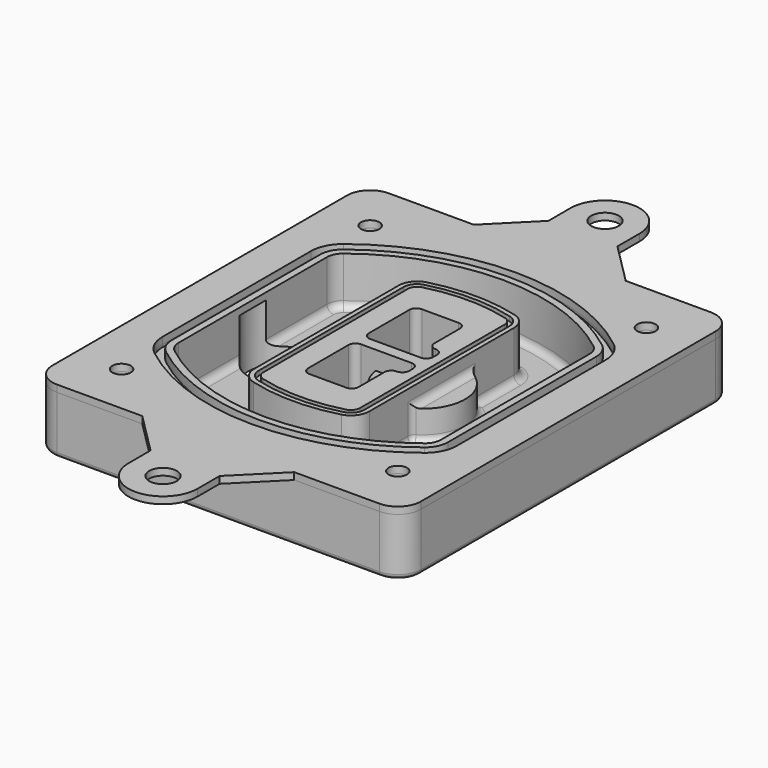
from build123d import *

# Parameters (mm, degrees)
F0_R      = 4
F1_DEPTH  = 25
F2_DEPTH  = 3
F3_DEPTH  = 1
F4_DEPTH  = 18
F6_DEPTH  = 21
F7_DEPTH  = 2
F9_DEPTH  = 20
F10_DEPTH = 16
F11_DEPTH = 25
F8_R      = 6
F8_R_2    = 4
F12_DEPTH = 6
F14_DEPTH = 9
F15_R     = 3
F16_R     = 2
F0_R_2    = 6
F17_DEPTH = 3


with BuildPart() as f1:
    # F0 (on Top) → F1 (new body)
    with BuildSketch(Plane.XY):
        with BuildLine():
            ThreePointArc((-80, -80), (-77.0710678119, -87.0710678119), (-70, -90))
            Line((-70, -90), (-33, -90))
            Line((-33, -90), (33, -90))
            Line((33, -90), (70, -90))
            ThreePointArc((70, -90), (77.0710678119, -87.0710678119), (80, -80))
            Line((80, -80), (80, 80))
            ThreePointArc((80, 80), (77.0710678119, 87.0710678119), (70, 90))
            Line((70, 90), (33, 90))
            Line((33, 90), (-33, 90))
            Line((-33, 90), (-70, 90))
            ThreePointArc((-70, 90), (-77.0710678119, 87.0710678119), (-80, 80))
            Line((-80, 80), (-80, -80))
        make_face()
        with Locations((-60, -67.5)):
            Circle(F0_R, mode=Mode.SUBTRACT)
        with Locations((60, -67.5)):
            Circle(F0_R, mode=Mode.SUBTRACT)
        with Locations((-60, 67.5)):
            Circle(F0_R, mode=Mode.SUBTRACT)
        with BuildLine():
            ThreePointArc((-64, 40.2934422872), (-62.5820384798, 46.4328484224), (-58.6153846154, 51.3286200352))
            ThreePointArc((-58.6153846154, 51.3286200352), (0, 71.5), (58.6153846154, 51.3286200352))
            ThreePointArc((58.6153846154, 51.3286200352), (62.5820384798, 46.4328484224), (64, 40.2934422872))
            Line((64, 40.2934422872), (64, -40.2934422872))
            ThreePointArc((64, -40.2934422872), (62.5820384798, -46.4328484224), (58.6153846154, -51.3286200352))
            ThreePointArc((58.6153846154, -51.3286200352), (0, -71.5), (-58.6153846154, -51.3286200352))
            ThreePointArc((-58.6153846154, -51.3286200352), (-62.5820384798, -46.4328484224), (-64, -40.2934422872))
            Line((-64, -40.2934422872), (-64, 40.2934422872))
        make_face(mode=Mode.SUBTRACT)
        with Locations((60, 67.5)):
            Circle(F0_R, mode=Mode.SUBTRACT)
        with BuildLine():
            ThreePointArc((58.6153846154, 51.3286200352), (0, 71.5), (-58.6153846154, 51.3286200352))
            ThreePointArc((-58.6153846154, 51.3286200352), (-62.5820384798, 46.4328484224), (-64, 40.2934422872))
            Line((-64, 40.2934422872), (-64, -40.2934422872))
            ThreePointArc((-64, -40.2934422872), (-62.5820384798, -46.4328484224), (-58.6153846154, -51.3286200352))
            ThreePointArc((-58.6153846154, -51.3286200352), (0, -71.5), (58.6153846154, -51.3286200352))
            ThreePointArc((58.6153846154, -51.3286200352), (62.5820384798, -46.4328484224), (64, -40.2934422872))
            Line((64, -40.2934422872), (64, 40.2934422872))
            ThreePointArc((64, 40.2934422872), (62.5820384798, 46.4328484224), (58.6153846154, 51.3286200352))
        make_face()
        with BuildLine():
            Line((-60, -40.2934422872), (-60, 40.2934422872))
            ThreePointArc((-60, 40.2934422872), (-58.9871703427, 44.6787323838), (-56.1538461538, 48.1757121072))
            ThreePointArc((-56.1538461538, 48.1757121072), (0, 67.5), (56.1538461538, 48.1757121072))
            ThreePointArc((56.1538461538, 48.1757121072), (58.9871703427, 44.6787323838), (60, 40.2934422872))
            Line((60, 40.2934422872), (60, -40.2934422872))
            ThreePointArc((60, -40.2934422872), (58.9871703427, -44.6787323838), (56.1538461538, -48.1757121072))
            ThreePointArc((56.1538461538, -48.1757121072), (0, -67.5), (-56.1538461538, -48.1757121072))
            ThreePointArc((-56.1538461538, -48.1757121072), (-58.9871703427, -44.6787323838), (-60, -40.2934422872))
        make_face(mode=Mode.SUBTRACT)
        with BuildLine():
            ThreePointArc((-56.1538461538, 48.1757121072), (-58.9871703427, 44.6787323838), (-60, 40.2934422872))
            Line((-60, 40.2934422872), (-60, -40.2934422872))
            ThreePointArc((-60, -40.2934422872), (-58.9871703427, -44.6787323838), (-56.1538461538, -48.1757121072))
            ThreePointArc((-56.1538461538, -48.1757121072), (0, -67.5), (56.1538461538, -48.1757121072))
            ThreePointArc((56.1538461538, -48.1757121072), (58.9871703427, -44.6787323838), (60, -40.2934422872))
            Line((60, -40.2934422872), (60, 40.2934422872))
            ThreePointArc((60, 40.2934422872), (58.9871703427, 44.6787323838), (56.1538461538, 48.1757121072))
            ThreePointArc((56.1538461538, 48.1757121072), (0, 67.5), (-56.1538461538, 48.1757121072))
        make_face()
        with BuildLine():
            ThreePointArc((54.3076923077, 45.8110311612), (56.2910192399, 43.3631453548), (57, 40.2934422872))
            Line((57, 40.2934422872), (57, -40.2934422872))
            ThreePointArc((57, -40.2934422872), (56.2910192399, -43.3631453548), (54.3076923077, -45.8110311612))
            ThreePointArc((54.3076923077, -45.8110311612), (0, -64.5), (-54.3076923077, -45.8110311612))
            ThreePointArc((-54.3076923077, -45.8110311612), (-56.2910192399, -43.3631453548), (-57, -40.2934422872))
            Line((-57, -40.2934422872), (-57, 40.2934422872))
            ThreePointArc((-57, 40.2934422872), (-56.2910192399, 43.3631453548), (-54.3076923077, 45.8110311612))
            ThreePointArc((-54.3076923077, 45.8110311612), (0, 64.5), (54.3076923077, 45.8110311612))
        make_face(mode=Mode.SUBTRACT)
        with BuildLine():
            Line((57, -40.2934422872), (57, 40.2934422872))
            ThreePointArc((57, 40.2934422872), (56.2910192399, 43.3631453548), (54.3076923077, 45.8110311612))
            ThreePointArc((54.3076923077, 45.8110311612), (0, 64.5), (-54.3076923077, 45.8110311612))
            ThreePointArc((-54.3076923077, 45.8110311612), (-56.2910192399, 43.3631453548), (-57, 40.2934422872))
            Line((-57, 40.2934422872), (-57, -40.2934422872))
            ThreePointArc((-57, -40.2934422872), (-56.2910192399, -43.3631453548), (-54.3076923077, -45.8110311612))
            ThreePointArc((-54.3076923077, -45.8110311612), (0, -64.5), (54.3076923077, -45.8110311612))
            ThreePointArc((54.3076923077, -45.8110311612), (56.2910192399, -43.3631453548), (57, -40.2934422872))
        make_face()
    extrude(amount=-F1_DEPTH)

    # F0 (on Top) → F2 (join)
    with BuildSketch(Plane.XY):
        with BuildLine():
            ThreePointArc((-56.1538461538, 48.1757121072), (-58.9871703427, 44.6787323838), (-60, 40.2934422872))
            Line((-60, 40.2934422872), (-60, -40.2934422872))
            ThreePointArc((-60, -40.2934422872), (-58.9871703427, -44.6787323838), (-56.1538461538, -48.1757121072))
            ThreePointArc((-56.1538461538, -48.1757121072), (0, -67.5), (56.1538461538, -48.1757121072))
            ThreePointArc((56.1538461538, -48.1757121072), (58.9871703427, -44.6787323838), (60, -40.2934422872))
            Line((60, -40.2934422872), (60, 40.2934422872))
            ThreePointArc((60, 40.2934422872), (58.9871703427, 44.6787323838), (56.1538461538, 48.1757121072))
            ThreePointArc((56.1538461538, 48.1757121072), (0, 67.5), (-56.1538461538, 48.1757121072))
        make_face()
        with BuildLine():
            ThreePointArc((54.3076923077, 45.8110311612), (56.2910192399, 43.3631453548), (57, 40.2934422872))
            Line((57, 40.2934422872), (57, -40.2934422872))
            ThreePointArc((57, -40.2934422872), (56.2910192399, -43.3631453548), (54.3076923077, -45.8110311612))
            ThreePointArc((54.3076923077, -45.8110311612), (0, -64.5), (-54.3076923077, -45.8110311612))
            ThreePointArc((-54.3076923077, -45.8110311612), (-56.2910192399, -43.3631453548), (-57, -40.2934422872))
            Line((-57, -40.2934422872), (-57, 40.2934422872))
            ThreePointArc((-57, 40.2934422872), (-56.2910192399, 43.3631453548), (-54.3076923077, 45.8110311612))
            ThreePointArc((-54.3076923077, 45.8110311612), (0, 64.5), (54.3076923077, 45.8110311612))
        make_face(mode=Mode.SUBTRACT)
    extrude(amount=F2_DEPTH)

    # F0 (on Top) → F3 (cut)
    with BuildSketch(Plane.XY):
        with BuildLine():
            ThreePointArc((58.6153846154, 51.3286200352), (0, 71.5), (-58.6153846154, 51.3286200352))
            ThreePointArc((-58.6153846154, 51.3286200352), (-62.5820384798, 46.4328484224), (-64, 40.2934422872))
            Line((-64, 40.2934422872), (-64, -40.2934422872))
            ThreePointArc((-64, -40.2934422872), (-62.5820384798, -46.4328484224), (-58.6153846154, -51.3286200352))
            ThreePointArc((-58.6153846154, -51.3286200352), (0, -71.5), (58.6153846154, -51.3286200352))
            ThreePointArc((58.6153846154, -51.3286200352), (62.5820384798, -46.4328484224), (64, -40.2934422872))
            Line((64, -40.2934422872), (64, 40.2934422872))
            ThreePointArc((64, 40.2934422872), (62.5820384798, 46.4328484224), (58.6153846154, 51.3286200352))
        make_face()
        with BuildLine():
            Line((-60, -40.2934422872), (-60, 40.2934422872))
            ThreePointArc((-60, 40.2934422872), (-58.9871703427, 44.6787323838), (-56.1538461538, 48.1757121072))
            ThreePointArc((-56.1538461538, 48.1757121072), (0, 67.5), (56.1538461538, 48.1757121072))
            ThreePointArc((56.1538461538, 48.1757121072), (58.9871703427, 44.6787323838), (60, 40.2934422872))
            Line((60, 40.2934422872), (60, -40.2934422872))
            ThreePointArc((60, -40.2934422872), (58.9871703427, -44.6787323838), (56.1538461538, -48.1757121072))
            ThreePointArc((56.1538461538, -48.1757121072), (0, -67.5), (-56.1538461538, -48.1757121072))
            ThreePointArc((-56.1538461538, -48.1757121072), (-58.9871703427, -44.6787323838), (-60, -40.2934422872))
        make_face(mode=Mode.SUBTRACT)
    extrude(amount=-F3_DEPTH, mode=Mode.SUBTRACT)

    # F0 (on Top) → F4 (cut)
    with BuildSketch(Plane.XY):
        with BuildLine():
            Line((57, -40.2934422872), (57, 40.2934422872))
            ThreePointArc((57, 40.2934422872), (56.2910192399, 43.3631453548), (54.3076923077, 45.8110311612))
            ThreePointArc((54.3076923077, 45.8110311612), (0, 64.5), (-54.3076923077, 45.8110311612))
            ThreePointArc((-54.3076923077, 45.8110311612), (-56.2910192399, 43.3631453548), (-57, 40.2934422872))
            Line((-57, 40.2934422872), (-57, -40.2934422872))
            ThreePointArc((-57, -40.2934422872), (-56.2910192399, -43.3631453548), (-54.3076923077, -45.8110311612))
            ThreePointArc((-54.3076923077, -45.8110311612), (0, -64.5), (54.3076923077, -45.8110311612))
            ThreePointArc((54.3076923077, -45.8110311612), (56.2910192399, -43.3631453548), (57, -40.2934422872))
        make_face()
    extrude(amount=-F4_DEPTH, mode=Mode.SUBTRACT)

    # F5 (on face) → F6 (join, through all)
    with BuildSketch(Plane.XY.offset(3)):
        with BuildLine():
            ThreePointArc((-25, -39.2465276821), (-23.3511545998, -44.1109737193), (-19.0842911877, -46.9702398883))
            ThreePointArc((-19.0842911877, -46.9702398883), (0, -49.5), (19.0842911877, -46.9702398883))
            ThreePointArc((19.0842911877, -46.9702398883), (23.3511545998, -44.1109737193), (25, -39.2465276821))
            Line((25, -39.2465276821), (25, 39.2465276821))
            ThreePointArc((25, 39.2465276821), (23.3511545998, 44.1109737193), (19.0842911877, 46.9702398883))
            ThreePointArc((19.0842911877, 46.9702398883), (0, 49.5), (-19.0842911877, 46.9702398883))
            ThreePointArc((-19.0842911877, 46.9702398883), (-23.3511545998, 44.1109737193), (-25, 39.2465276821))
            Line((-25, 39.2465276821), (-25, -39.2465276821))
        make_face()
        with BuildLine():
            ThreePointArc((18.5632183908, 45.0393118368), (21.7633659499, 42.89486221), (23, 39.2465276821))
            Line((23, 39.2465276821), (23, -39.2465276821))
            ThreePointArc((23, -39.2465276821), (21.7633659499, -42.89486221), (18.5632183908, -45.0393118368))
            ThreePointArc((18.5632183908, -45.0393118368), (0, -47.5), (-18.5632183908, -45.0393118368))
            ThreePointArc((-18.5632183908, -45.0393118368), (-21.7633659499, -42.89486221), (-23, -39.2465276821))
            Line((-23, -39.2465276821), (-23, 39.2465276821))
            ThreePointArc((-23, 39.2465276821), (-21.7633659499, 42.89486221), (-18.5632183908, 45.0393118368))
            ThreePointArc((-18.5632183908, 45.0393118368), (0, 47.5), (18.5632183908, 45.0393118368))
        make_face(mode=Mode.SUBTRACT)
        with BuildLine():
            Line((23, -39.2465276821), (23, 39.2465276821))
            ThreePointArc((23, 39.2465276821), (21.7633659499, 42.89486221), (18.5632183908, 45.0393118368))
            ThreePointArc((18.5632183908, 45.0393118368), (0, 47.5), (-18.5632183908, 45.0393118368))
            ThreePointArc((-18.5632183908, 45.0393118368), (-21.7633659499, 42.89486221), (-23, 39.2465276821))
            Line((-23, 39.2465276821), (-23, -39.2465276821))
            ThreePointArc((-23, -39.2465276821), (-21.7633659499, -42.89486221), (-18.5632183908, -45.0393118368))
            ThreePointArc((-18.5632183908, -45.0393118368), (0, -47.5), (18.5632183908, -45.0393118368))
            ThreePointArc((18.5632183908, -45.0393118368), (21.7633659499, -42.89486221), (23, -39.2465276821))
        make_face()
        with BuildLine():
            ThreePointArc((18.0421455939, 43.1083837852), (20.1755772999, 41.6787507007), (21, 39.2465276821))
            Line((21, 39.2465276821), (21, -39.2465276821))
            ThreePointArc((21, -39.2465276821), (20.1755772999, -41.6787507007), (18.0421455939, -43.1083837852))
            ThreePointArc((18.0421455939, -43.1083837852), (0, -45.5), (-18.0421455939, -43.1083837852))
            ThreePointArc((-18.0421455939, -43.1083837852), (-20.1755772999, -41.6787507007), (-21, -39.2465276821))
            Line((-21, -39.2465276821), (-21, 39.2465276821))
            ThreePointArc((-21, 39.2465276821), (-20.1755772999, 41.6787507007), (-18.0421455939, 43.1083837852))
            ThreePointArc((-18.0421455939, 43.1083837852), (0, 45.5), (18.0421455939, 43.1083837852))
        make_face(mode=Mode.SUBTRACT)
        with BuildLine():
            Line((21, -39.2465276821), (21, 39.2465276821))
            ThreePointArc((21, 39.2465276821), (20.1755772999, 41.6787507007), (18.0421455939, 43.1083837852))
            ThreePointArc((18.0421455939, 43.1083837852), (0, 45.5), (-18.0421455939, 43.1083837852))
            ThreePointArc((-18.0421455939, 43.1083837852), (-20.1755772999, 41.6787507007), (-21, 39.2465276821))
            Line((-21, 39.2465276821), (-21, -39.2465276821))
            ThreePointArc((-21, -39.2465276821), (-20.1755772999, -41.6787507007), (-18.0421455939, -43.1083837852))
            ThreePointArc((-18.0421455939, -43.1083837852), (0, -45.5), (18.0421455939, -43.1083837852))
            ThreePointArc((18.0421455939, -43.1083837852), (20.1755772999, -41.6787507007), (21, -39.2465276821))
        make_face()
        with BuildLine():
            Line((-8, -2.5), (14, -2.5))
            ThreePointArc((14, -2.5), (16.1213203436, -3.3786796564), (17, -5.5))
            Line((17, -5.5), (17, -7.5))
            ThreePointArc((17, -7.5), (16.1213203436, -9.6213203436), (14, -10.5))
            ThreePointArc((14, -10.5), (11.8786796564, -11.3786796564), (11, -13.5))
            Line((11, -13.5), (11, -27.5))
            ThreePointArc((11, -27.5), (10.1213203436, -29.6213203436), (8, -30.5))
            Line((8, -30.5), (-8, -30.5))
            ThreePointArc((-8, -30.5), (-10.1213203436, -29.6213203436), (-11, -27.5))
            Line((-11, -27.5), (-11, -5.5))
            ThreePointArc((-11, -5.5), (-10.1213203436, -3.3786796564), (-8, -2.5))
        make_face(mode=Mode.SUBTRACT)
        with BuildLine():
            ThreePointArc((-8, 2.5), (-10.1213203436, 3.3786796564), (-11, 5.5))
            Line((-11, 5.5), (-11, 27.5))
            ThreePointArc((-11, 27.5), (-10.1213203436, 29.6213203436), (-8, 30.5))
            Line((-8, 30.5), (8, 30.5))
            ThreePointArc((8, 30.5), (10.1213203436, 29.6213203436), (11, 27.5))
            Line((11, 27.5), (11, 13.5))
            ThreePointArc((11, 13.5), (11.8786796564, 11.3786796564), (14, 10.5))
            ThreePointArc((14, 10.5), (16.1213203436, 9.6213203436), (17, 7.5))
            Line((17, 7.5), (17, 5.5))
            ThreePointArc((17, 5.5), (16.1213203436, 3.3786796564), (14, 2.5))
            Line((14, 2.5), (-8, 2.5))
        make_face(mode=Mode.SUBTRACT)
    extrude(amount=-F6_DEPTH)

    # F5 (on face) → F7 (cut)
    with BuildSketch(Plane.XY.offset(3)):
        with BuildLine():
            Line((23, -39.2465276821), (23, 39.2465276821))
            ThreePointArc((23, 39.2465276821), (21.7633659499, 42.89486221), (18.5632183908, 45.0393118368))
            ThreePointArc((18.5632183908, 45.0393118368), (0, 47.5), (-18.5632183908, 45.0393118368))
            ThreePointArc((-18.5632183908, 45.0393118368), (-21.7633659499, 42.89486221), (-23, 39.2465276821))
            Line((-23, 39.2465276821), (-23, -39.2465276821))
            ThreePointArc((-23, -39.2465276821), (-21.7633659499, -42.89486221), (-18.5632183908, -45.0393118368))
            ThreePointArc((-18.5632183908, -45.0393118368), (0, -47.5), (18.5632183908, -45.0393118368))
            ThreePointArc((18.5632183908, -45.0393118368), (21.7633659499, -42.89486221), (23, -39.2465276821))
        make_face()
        with BuildLine():
            ThreePointArc((18.0421455939, 43.1083837852), (20.1755772999, 41.6787507007), (21, 39.2465276821))
            Line((21, 39.2465276821), (21, -39.2465276821))
            ThreePointArc((21, -39.2465276821), (20.1755772999, -41.6787507007), (18.0421455939, -43.1083837852))
            ThreePointArc((18.0421455939, -43.1083837852), (0, -45.5), (-18.0421455939, -43.1083837852))
            ThreePointArc((-18.0421455939, -43.1083837852), (-20.1755772999, -41.6787507007), (-21, -39.2465276821))
            Line((-21, -39.2465276821), (-21, 39.2465276821))
            ThreePointArc((-21, 39.2465276821), (-20.1755772999, 41.6787507007), (-18.0421455939, 43.1083837852))
            ThreePointArc((-18.0421455939, 43.1083837852), (0, 45.5), (18.0421455939, 43.1083837852))
        make_face(mode=Mode.SUBTRACT)
    extrude(amount=-F7_DEPTH, mode=Mode.SUBTRACT)

    # F8 (on face) → F9 (join)
    with BuildSketch(Plane(origin=(0, 0, -25), x_dir=(1, 0, 0), z_dir=(0, 0, -1))):
        with BuildLine():
            ThreePointArc((3.28842436, 0), (16.7567035675, 13.4682792075), (30.224982775, 0))
            Line((30.224982775, 0), (35.224982775, 0))
            ThreePointArc((35.224982775, 0), (16.7567035675, 18.4682792075), (-1.71157564, 0))
            Line((-1.71157564, 0), (3.28842436, 0))
        make_face()
        with BuildLine():
            Line((3.28842436, 0), (30.224982775, 0))
            ThreePointArc((30.224982775, 0), (16.7567035675, 13.4682792075), (3.28842436, 0))
        make_face()
        with BuildLine():
            ThreePointArc((3.28842436, 0), (16.7567035675, -13.4682792075), (30.224982775, 0))
            Line((30.224982775, 0), (3.28842436, 0))
        make_face()
        with BuildLine():
            Line((35.224982775, 0), (30.224982775, 0))
            ThreePointArc((30.224982775, 0), (16.7567035675, -13.4682792075), (3.28842436, 0))
            Line((3.28842436, 0), (-1.71157564, 0))
            ThreePointArc((-1.71157564, 0), (16.7567035675, -18.4682792075), (35.224982775, 0))
        make_face()
    extrude(amount=-F9_DEPTH)

    # F8 (on face) → F10 (cut)
    with BuildSketch(Plane(origin=(0, 0, -25), x_dir=(1, 0, 0), z_dir=(0, 0, -1))):
        with BuildLine():
            Line((3.28842436, 0), (30.224982775, 0))
            ThreePointArc((30.224982775, 0), (16.7567035675, 13.4682792075), (3.28842436, 0))
        make_face()
        with BuildLine():
            ThreePointArc((3.28842436, 0), (16.7567035675, -13.4682792075), (30.224982775, 0))
            Line((30.224982775, 0), (3.28842436, 0))
        make_face()
    extrude(amount=-F10_DEPTH, mode=Mode.SUBTRACT)

    # F8 (on face) → F11 (cut)
    with BuildSketch(Plane(origin=(0, 0, -25), x_dir=(1, 0, 0), z_dir=(0, 0, -1))):
        with BuildLine():
            Line((-59.0318229325, 0), (-32.0952645175, 0))
            ThreePointArc((-32.0952645175, 0), (-45.563543725, 13.4682792075), (-59.0318229325, 0))
        make_face()
        with BuildLine():
            ThreePointArc((-59.0318229325, 0), (-45.563543725, -13.4682792075), (-32.0952645175, 0))
            Line((-32.0952645175, 0), (-59.0318229325, 0))
        make_face()
    extrude(amount=-F11_DEPTH, mode=Mode.SUBTRACT)

    # F8 (on face) → F12 (cut)
    with BuildSketch(Plane(origin=(0, 0, -25), x_dir=(1, 0, 0), z_dir=(0, 0, -1))):
        with Locations((60, -67.5)):
            Circle(F8_R)
        with Locations((60, -67.5)):
            Circle(F8_R_2, mode=Mode.SUBTRACT)
        with Locations((-60, -67.5)):
            Circle(F8_R)
        with Locations((-60, -67.5)):
            Circle(F8_R_2, mode=Mode.SUBTRACT)
        with Locations((-60, 67.5)):
            Circle(F8_R)
        with Locations((-60, 67.5)):
            Circle(F8_R_2, mode=Mode.SUBTRACT)
        with Locations((60, 67.5)):
            Circle(F8_R)
        with Locations((60, 67.5)):
            Circle(F8_R_2, mode=Mode.SUBTRACT)
    extrude(amount=-F12_DEPTH, mode=Mode.SUBTRACT)

    # F13 (on face) → F14 (cut, through all)
    with BuildSketch(Plane(origin=(0, 0, -9), x_dir=(1, 0, 0), z_dir=(0, 0, -1))):
        with BuildLine():
            Line((11, 13.5), (11, 17.5481537753))
            ThreePointArc((11, 17.5481537753), (2.5696536419, 11.8239143813), (-1.5415842455, 2.5))
            Line((-1.5415842455, 2.5), (3.5224848595, 2.5))
            ThreePointArc((3.5224848595, 2.5), (6.1857188154, 8.3455872281), (11.2536447004, 12.2927168648))
            ThreePointArc((11.2536447004, 12.2927168648), (11.0640958889, 12.8831798879), (11, 13.5))
        make_face()
        with BuildLine():
            ThreePointArc((11.2536447004, -12.2927168648), (6.1857188154, -8.3455872281), (3.5224848595, -2.5))
            Line((3.5224848595, -2.5), (-1.5415842455, -2.5))
            ThreePointArc((-1.5415842455, -2.5), (2.5696536419, -11.8239143813), (11, -17.5481537753))
            Line((11, -17.5481537753), (11, -13.5))
            ThreePointArc((11, -13.5), (11.0640958889, -12.8831798879), (11.2536447004, -12.2927168648))
        make_face()
        with BuildLine():
            ThreePointArc((11.2536447004, 12.2927168648), (6.1857188154, 8.3455872281), (3.5224848595, 2.5))
            Line((3.5224848595, 2.5), (14, 2.5))
            ThreePointArc((14, 2.5), (16.1213203436, 3.3786796564), (17, 5.5))
            Line((17, 5.5), (17, 7.5))
            ThreePointArc((17, 7.5), (16.1213203436, 9.6213203436), (14, 10.5))
            ThreePointArc((14, 10.5), (12.3601599782, 10.9878446101), (11.2536447004, 12.2927168648))
        make_face()
        with BuildLine():
            Line((14, -2.5), (3.5224848595, -2.5))
            ThreePointArc((3.5224848595, -2.5), (6.1857188154, -8.3455872281), (11.2536447004, -12.2927168648))
            ThreePointArc((11.2536447004, -12.2927168648), (12.3601599782, -10.9878446101), (14, -10.5))
            ThreePointArc((14, -10.5), (16.1213203436, -9.6213203436), (17, -7.5))
            Line((17, -7.5), (17, -5.5))
            ThreePointArc((17, -5.5), (16.1213203436, -3.3786796564), (14, -2.5))
        make_face()
    extrude(amount=F14_DEPTH, mode=Mode.SUBTRACT)

    # F15
    f15_edges = [f1.edges().sort_by_distance(p)[0] for p in [
        (-57, -23.703476, -18),
        (-57, 23.703476, -18),
        (25, 0, -5),
        (25, 16.526506, -11.5),
        (25, -16.526506, -11.5),
        (25, -27.886517, -18),
        (35.224983, 0, -18),
    ]]
    fillet(f15_edges, radius=F15_R)

    # F16
    f16_edges = [f1.edges().sort_by_distance(p)[0] for p in [
        (0, -90, -25),
    ]]
    fillet(f16_edges, radius=F16_R)


with BuildPart() as f17:
    # F0 (on Top) → F17 (new body, through all)
    with BuildSketch(Plane.XY):
        with BuildLine():
            ThreePointArc((-80, -80), (-77.0710678119, -87.0710678119), (-70, -90))
            Line((-70, -90), (-33, -90))
            Line((-33, -90), (33, -90))
            Line((33, -90), (70, -90))
            ThreePointArc((70, -90), (77.0710678119, -87.0710678119), (80, -80))
            Line((80, -80), (80, 80))
            ThreePointArc((80, 80), (77.0710678119, 87.0710678119), (70, 90))
            Line((70, 90), (33, 90))
            Line((33, 90), (-33, 90))
            Line((-33, 90), (-70, 90))
            ThreePointArc((-70, 90), (-77.0710678119, 87.0710678119), (-80, 80))
            Line((-80, 80), (-80, -80))
        make_face()
        with Locations((-60, -67.5)):
            Circle(F0_R, mode=Mode.SUBTRACT)
        with Locations((60, -67.5)):
            Circle(F0_R, mode=Mode.SUBTRACT)
        with Locations((-60, 67.5)):
            Circle(F0_R, mode=Mode.SUBTRACT)
        with BuildLine():
            ThreePointArc((-64, 40.2934422872), (-62.5820384798, 46.4328484224), (-58.6153846154, 51.3286200352))
            ThreePointArc((-58.6153846154, 51.3286200352), (0, 71.5), (58.6153846154, 51.3286200352))
            ThreePointArc((58.6153846154, 51.3286200352), (62.5820384798, 46.4328484224), (64, 40.2934422872))
            Line((64, 40.2934422872), (64, -40.2934422872))
            ThreePointArc((64, -40.2934422872), (62.5820384798, -46.4328484224), (58.6153846154, -51.3286200352))
            ThreePointArc((58.6153846154, -51.3286200352), (0, -71.5), (-58.6153846154, -51.3286200352))
            ThreePointArc((-58.6153846154, -51.3286200352), (-62.5820384798, -46.4328484224), (-64, -40.2934422872))
            Line((-64, -40.2934422872), (-64, 40.2934422872))
        make_face(mode=Mode.SUBTRACT)
        with Locations((60, 67.5)):
            Circle(F0_R, mode=Mode.SUBTRACT)
        with BuildLine():
            Line((33, -90), (-33, -90))
            Line((-33, -90), (-15, -108))
            Line((-15, -108), (-15, -120))
            ThreePointArc((-15, -120), (0, -135), (15, -120))
            Line((15, -120), (15, -108))
            Line((15, -108), (33, -90))
        make_face()
        with Locations((0, -120)):
            Circle(F0_R_2, mode=Mode.SUBTRACT)
        with BuildLine():
            Line((-15, 108), (-33, 90))
            Line((-33, 90), (33, 90))
            Line((33, 90), (15, 108))
            Line((15, 108), (15, 120))
            ThreePointArc((15, 120), (0, 135), (-15, 120))
            Line((-15, 120), (-15, 108))
        make_face()
        with Locations((0, 120)):
            Circle(F0_R_2, mode=Mode.SUBTRACT)
    extrude(amount=F17_DEPTH)


solid = Compound([f1.part, f17.part])
